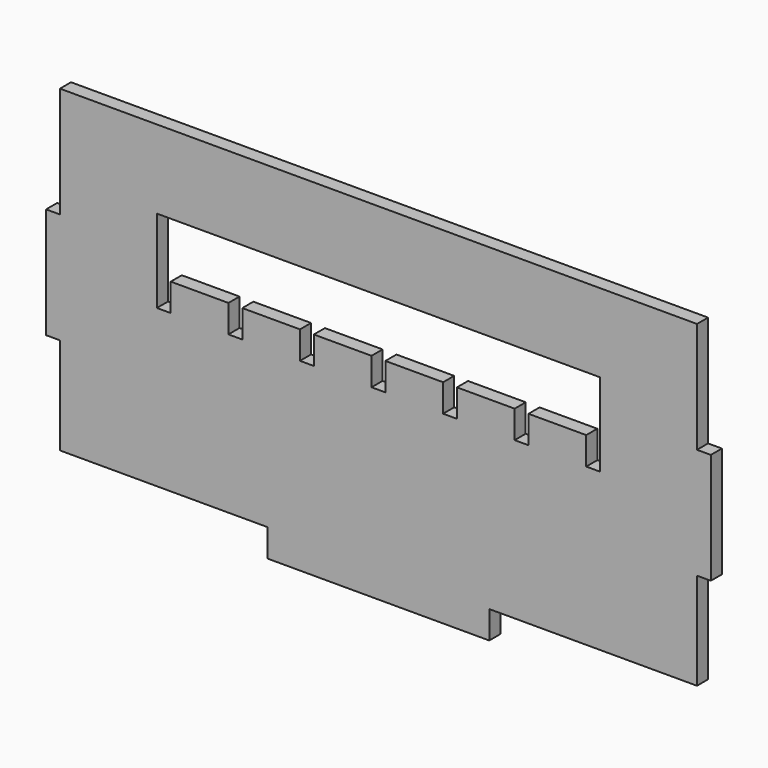
from build123d import *

# Parameters (mm, degrees)
F0_W     = 19.05
F0_H     = 152.4
F0_W_2   = 304.8
F0_H_2   = 38.1
F1_DEPTH = 19.05


# Not quite as in the source:
# - a feature names something its author has since deleted; it is built from what else it names


with BuildPart() as f1:
    # F0 (on Front) → F1 (new body)
    with BuildSketch(Plane.XZ):
        Polygon((438.15, 219.075), (-438.15, 219.075), (-438.15, 66.675), (-438.15, -85.725), (-438.15, -219.075), (-152.4, -219.075), (152.4, -219.075), (438.15, -219.075), (438.15, -85.725), (438.15, 66.675), align=None)
        Polygon((-304.8, 111.125), (304.8, 111.125), (304.8, 34.925), (304.8, -3.175), (285.75, -3.175), (285.75, 34.925), (206.375, 34.925), (206.375, -3.175), (187.325, -3.175), (187.325, 34.925), (107.95, 34.925), (107.95, -3.175), (88.9, -3.175), (88.9, 34.925), (9.525, 34.925), (9.525, -3.175), (-9.525, -3.175), (-9.525, 34.925), (-88.9, 34.925), (-88.9, -3.175), (-107.95, -3.175), (-107.95, 34.925), (-187.325, 34.925), (-187.325, -3.175), (-206.375, -3.175), (-206.375, 34.925), (-285.75, 34.925), (-285.75, -3.175), (-304.8, -3.175), (-304.8, 34.925), align=None, mode=Mode.SUBTRACT)
        with Locations((-447.675, -9.525)):
            Rectangle(F0_W, F0_H)
        with Locations((0, -238.125)):
            Rectangle(F0_W_2, F0_H_2)
        with Locations((447.675, -9.525)):
            Rectangle(F0_W, F0_H)
    extrude(amount=F1_DEPTH)


solid = f1.part
